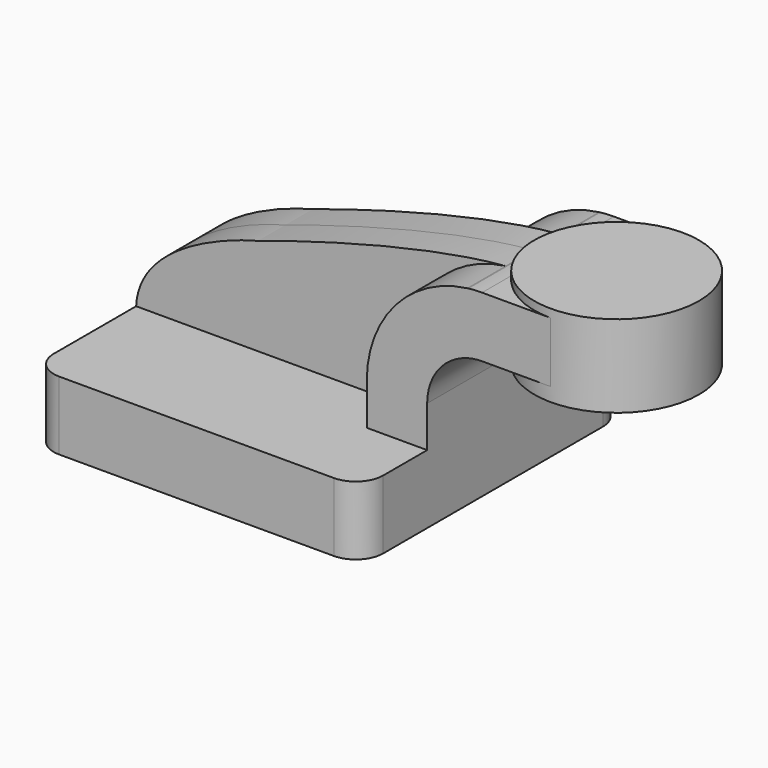
from build123d import *

# Parameters (mm, degrees)
F1_DEPTH = 60
F2_DEPTH = 30
F3_DEPTH = 12.5
F5_R     = 10


# Not quite as in the source:
# - a feature names something its author has since deleted; it is built from what else it names


with BuildPart() as f1:
    # F0 (on Front) → F1 (new body, symmetric)
    with BuildSketch(Plane.XZ):
        Polygon((-60, 12.5), (-60, -12.5), (60, -12.5), (60, 12.5), (38, 12.5), align=None)
    extrude(amount=F1_DEPTH, both=True)

    # F0 (on Front) → F2 (join, symmetric)
    with BuildSketch(Plane.XZ):
        with BuildLine():
            Line((38, 12.5), (60, 12.5))
            Line((60, 12.5), (60, 27.5))
            ThreePointArc((60, 27.5), (64.1886116992, 39.7474487139), (75, 46.864916731))
            Line((75, 46.864916731), (75, 69.1849707307))
            add(Edge.make_bspline(
                [(74.6086884092, 69.1525360492), (74.7393390429, 69.163538875), (74.8697772932, 69.1743509337), (75, 69.1849707307)],
                knots=[0.9728827871, 0.9728827871, 0.9728827871, 0.9728827871, 0.9748058763, 0.9748058763, 0.9748058763, 0.9748058763], degree=3))
            ThreePointArc((74.6086884092, 69.1525360492), (48.4529313025, 55.2269265623), (38, 27.5))
            Line((38, 27.5), (38, 12.5))
        make_face()
        with BuildLine():
            ThreePointArc((80, 69.5), (77.4955434529, 69.425263236), (75, 69.201318924))
            Line((75, 69.201318924), (75, 69.1849707307))
            add(Edge.make_bspline(
                [(75, 69.1849707307), (76.7060295657, 69.324099213), (78.3750648422, 69.4302293108), (80, 69.5)],
                knots=[0.9748058763, 0.9748058763, 0.9748058763, 0.9748058763, 1, 1, 1, 1], degree=3))
        make_face()
        with BuildLine():
            add(Edge.make_bspline(
                [(75, 69.1849707307), (76.7060295657, 69.324099213), (78.3750648422, 69.4302293108), (80, 69.5)],
                knots=[0.9748058763, 0.9748058763, 0.9748058763, 0.9748058763, 1, 1, 1, 1], degree=3))
            Line((75, 69.1849707307), (75, 46.864916731))
            ThreePointArc((75, 46.864916731), (77.4799141503, 47.3405939253), (80, 47.5))
            Line((80, 47.5), (105, 47.5))
            Line((105, 47.5), (105, 69.5))
            Line((105, 69.5), (80, 69.5))
        make_face()
    extrude(amount=F2_DEPTH, both=True)

    # F0 (on Front) → F3 (join, symmetric)
    with BuildSketch(Plane.XZ):
        with BuildLine():
            add(Edge.make_bspline(
                [(-60, 12.5), (-58.7895740645, 37.710647482), (-15.7147551824, 47.8502400891), (-15.7294783827, 47.857399648), (37.8509932243, 66.056963491), (74.6086884092, 69.1525360492)],
                knots=[0, 0, 0, 0, 0.4317155285, 0.4318343159, 0.9728827871, 0.9728827871, 0.9728827871, 0.9728827871], degree=3))
            Line((-60, 12.5), (38, 12.5))
            Line((38, 12.5), (38, 27.5))
            ThreePointArc((38, 27.5), (48.4529313025, 55.2269265623), (74.6086884092, 69.1525360492))
        make_face()
    extrude(amount=F3_DEPTH, both=True)

    # F0 (on Front) → F4 (revolve)
    with BuildSketch(Plane.XZ):
        Polygon((135, 72.5), (105, 72.5), (105, 69.5), (105, 47.5), (105, 42.5), (135, 42.5), align=None)
    revolve(axis=Axis((105, 0, 58.5), (0, 0, 1)))

    # F5
    f5_edges = [f1.edges().sort_by_distance(p)[0] for p in [
        (-60, -60, 0),
        (60, -60, 0),
        (60, 60, 0),
        (-60, 60, 0),
    ]]
    fillet(f5_edges, radius=F5_R)


solid = f1.part
